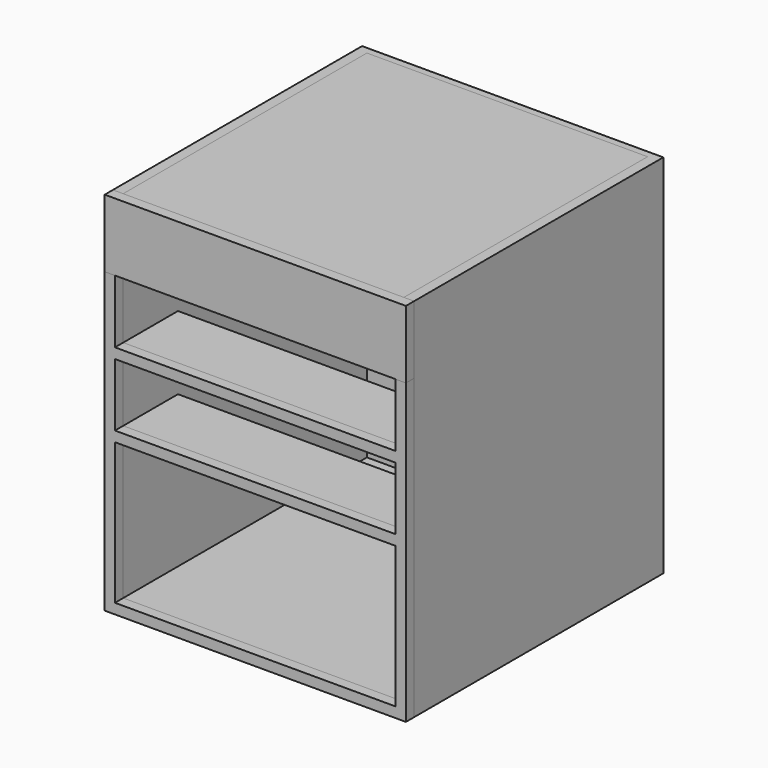
from build123d import *

# Parameters (mm, degrees)
F4_W      = 19.05
F4_H      = 565.15
F5_DEPTH  = 679.45
F6_W      = 520.7
F6_H      = 565.15
F7_DEPTH  = 19.05
F8_W      = 520.7
F8_H      = 565.15
F9_DEPTH  = 19.05
F10_W     = 558.8
F10_H     = 135.73125
F11_DEPTH = 19.05
F12_W     = 520.7
F12_H     = 19.05
F13_DEPTH = 565.15
F15_DEPTH = 19.05
F19_W     = 127
F19_H     = 19.05
F20_DEPTH = 520.7
F21_W     = 558.8
F21_H     = 125.8744746447
F22_DEPTH = 19.05
F23_W     = 263.5020315647
F23_H     = 73.9188790321
F24_DEPTH = 19.05
F25_W     = 520.7
F25_H     = 116.84
F25_H_2   = 19.05
F26_DEPTH = 19.05


# Not quite as in the source:
# - a variable given as a bare number and used for a length is read in inches; the dataset says mm whatever the document's units were


with BuildPart() as f5:
    # F4 (on Top) → F5 (new body)
    with BuildSketch(Plane.XY):
        Polygon((558.8, 577.85), (0, 577.85), (0, 565.15), (19.05, 565.15), (539.75, 565.15), (558.8, 565.15), align=None)
        with Locations((9.525, 282.575)):
            Rectangle(F4_W, F4_H)
        with Locations((549.275, 282.575)):
            Rectangle(F4_W, F4_H)
    extrude(amount=-F5_DEPTH)


with BuildPart() as f7:
    # F6 (on Top) → F7 (new body)
    with BuildSketch(Plane.XY):
        with Locations((279.4, 282.575)):
            Rectangle(F6_W, F6_H)
    extrude(amount=-F7_DEPTH)


with BuildPart() as f9:
    # F8 (on face) → F9 (new body)
    with BuildSketch(Plane(origin=(0, 0, -679.45), x_dir=(1, 0, 0), z_dir=(0, 0, -1))):
        with Locations((279.4, -282.575)):
            Rectangle(F8_W, F8_H)
    extrude(amount=-F9_DEPTH)


with BuildPart() as f11:
    # F10 (on face) → F11 (new body)
    with BuildSketch(Plane.XZ):
        with Locations((279.4, -67.865625)):
            Rectangle(F10_W, F10_H)
    extrude(amount=F11_DEPTH)


with BuildPart() as f13:
    # F12 (on face) → F13 (new body)
    with BuildSketch(Plane.XZ.offset(-565.15)):
        with Locations((279.4, -349.25)):
            Rectangle(F12_W, F12_H)
    extrude(amount=F13_DEPTH)


with BuildPart() as f15:
    # F14 (on face) → F15 (new body)
    with BuildSketch(Plane.XZ):
        Polygon((558.8, -135.73125), (539.75, -135.73125), (539.75, -339.725), (539.75, -358.775), (539.75, -660.4), (539.75, -679.45), (558.8, -679.45), align=None)
        Polygon((539.75, -358.775), (539.75, -339.725), (19.05, -339.725), (19.05, -135.73125), (0, -135.73125), (0, -679.45), (19.05, -679.45), (539.75, -679.45), (539.75, -660.4), (19.05, -660.4), (19.05, -358.775), align=None)
    extrude(amount=F15_DEPTH)


with BuildPart() as f20:
    # F19 (on face) → F20 (new body, through all)
    with BuildSketch(Plane.YZ.offset(19.05)):
        with Locations((501.65, -116.84)):
            Rectangle(F19_W, F19_H)
    extrude(amount=F20_DEPTH)


with BuildPart() as f20b:
    # F19 (on face) → F20, piece 2 (new body, through all)
    with BuildSketch(Plane.YZ.offset(19.05)):
        with Locations((63.5, -116.84)):
            Rectangle(F19_W, F19_H)
    extrude(amount=F20_DEPTH)


with BuildPart() as f20c:
    # F19 (on face) → F20, piece 3 (new body, through all)
    with BuildSketch(Plane.YZ.offset(19.05)):
        with Locations((63.5, -252.73)):
            Rectangle(F19_W, F19_H)
    extrude(amount=F20_DEPTH)


with BuildPart() as f20d:
    # F19 (on face) → F20, piece 4 (new body, through all)
    with BuildSketch(Plane.YZ.offset(19.05)):
        with Locations((501.65, -252.73)):
            Rectangle(F19_W, F19_H)
    extrude(amount=F20_DEPTH)


with BuildPart() as f20e:
    # F19 (on face) → F20, piece 5 (new body, through all)
    with BuildSketch(Plane.YZ.offset(19.05)):
        with Locations((63.5, -388.62)):
            Rectangle(F19_W, F19_H)
    extrude(amount=F20_DEPTH)


with BuildPart() as f20f:
    # F19 (on face) → F20, piece 6 (new body, through all)
    with BuildSketch(Plane.YZ.offset(19.05)):
        with Locations((501.65, -388.62)):
            Rectangle(F19_W, F19_H)
    extrude(amount=F20_DEPTH)


with BuildPart() as f22:
    # F21 (on Front) → F22 (new body)
    with BuildSketch(Plane.XZ):
        with Locations((279.4, -62.9372373223)):
            Rectangle(F21_W, F21_H)
    extrude(amount=F22_DEPTH)


with BuildPart() as f24:
    # F23 (on Front) → F24 (new body)
    with BuildSketch(Plane.XZ):
        with Locations((339.2337411642, -197.9473680258)):
            Rectangle(F23_W, F23_H)
    extrude(amount=F24_DEPTH)


with BuildPart() as f26:
    # F25 (on face) → F26 (new body)
    with BuildSketch(Plane.XZ):
        Polygon((19.05, -125.8744746447), (0, -125.8744746447), (0, -679.45), (19.05, -679.45), (19.05, -660.4), (19.05, -398.145), (539.75, -398.145), (539.75, -660.4), (539.75, -679.45), (558.8, -679.45), (558.8, -125.8744746447), (539.75, -125.8744746447), (539.75, -243.205), (19.05, -243.205), align=None)
        with Locations((279.4, -320.675)):
            Rectangle(F25_W, F25_H, mode=Mode.SUBTRACT)
        with Locations((279.4, -669.925)):
            Rectangle(F25_W, F25_H_2)
    extrude(amount=F26_DEPTH)


solid = Compound([f5.part, f7.part, f9.part, f20.part, f20b.part, f20c.part, f20d.part, f20e.part, f20f.part, f22.part, f26.part])
